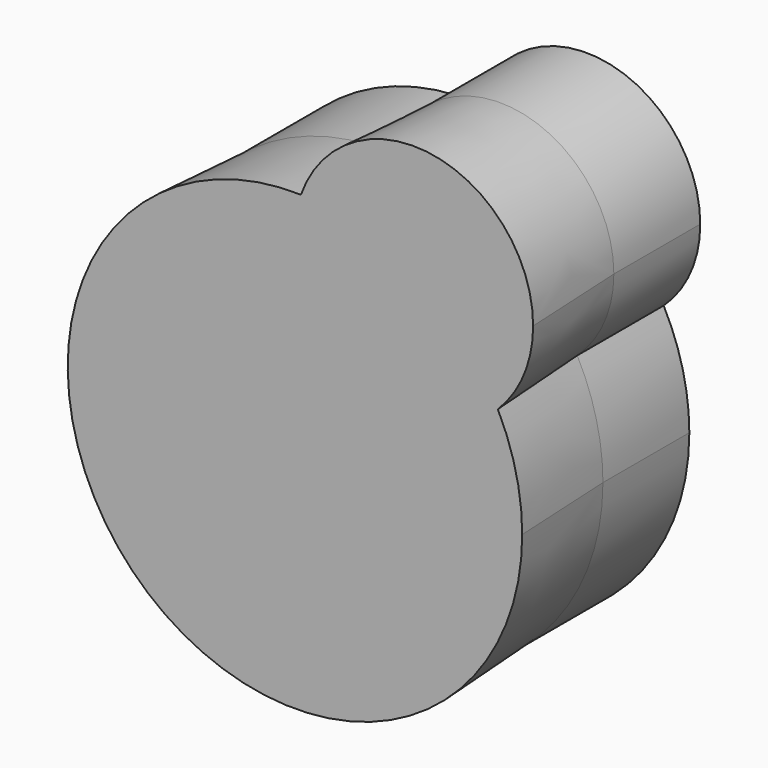
from build123d import *

# Parameters (mm, degrees)
F1_DEPTH               = 25.4
F2_DEPTH               = 25.4
DRAFT_F2_DRAFTED_ANGLE = -3


# Not quite as in the source:
# - an extrude with a draft is written as a straight extrude whose walls are then drafted


with BuildPart() as f1:
    # F0 (on Front) → F1 (new body)
    with BuildSketch(Plane.XZ):
        with BuildLine():
            ThreePointArc((2.3443913979, 52.06451709), (-37.672227148, -36.0140724239), (52.1172726727, 0))
            ThreePointArc((52.1172726727, 0), (50.5851100924, 12.5441917946), (46.0787084997, 24.350826143))
            ThreePointArc((46.0787084997, 24.350826143), (13.5580091507, 21.3955720513), (2.3443913979, 52.06451709))
        make_face()
        with BuildLine():
            ThreePointArc((2.3443913979, 52.06451709), (27.8964391527, 44.0227077023), (46.0787084997, 24.350826143))
            ThreePointArc((46.0787084997, 24.350826143), (52.438627232, 33.2868403889), (54.684082623, 44.0227077023))
            ThreePointArc((54.684082623, 44.0227077023), (31.9645282311, 70.4996503872), (2.3443913979, 52.06451709))
        make_face()
        with BuildLine():
            ThreePointArc((2.3443913979, 52.06451709), (13.5580091507, 21.3955720513), (46.0787084997, 24.350826143))
            ThreePointArc((46.0787084997, 24.350826143), (27.8964391527, 44.0227077023), (2.3443913979, 52.06451709))
        make_face()
    extrude(amount=F1_DEPTH)


with BuildPart() as f2_drafted:
    # F2 (new): a face of the model
    f2_faces = [f1.part.faces().sort_by_distance(p)[0] for p in [
        (4.2536608334, -25.4, 6.7126010781),
    ]]
    extrude(f2_faces, amount=F2_DEPTH)

    # draft_F2_drafted
    draft_f2_drafted_walls = [f2_drafted.faces().sort_by_distance(p)[0] for p in [
        (-27.8964391527, -42.3333333333, -44.0227077023),
        (42.2348691547, -42.3333333333, 66.6498433533),
    ]]
    draft(draft_f2_drafted_walls, neutral_plane=Plane(origin=(4.2536608334, -25.4, 6.7126010781), x_dir=(1, 0, 0), z_dir=(0, -1, 0)), angle=DRAFT_F2_DRAFTED_ANGLE)


with BuildPart() as f1_1:
    add(f1.part)

    # join_F2_drafted: union F2_drafted
    add(f2_drafted.part)


solid = f1_1.part
